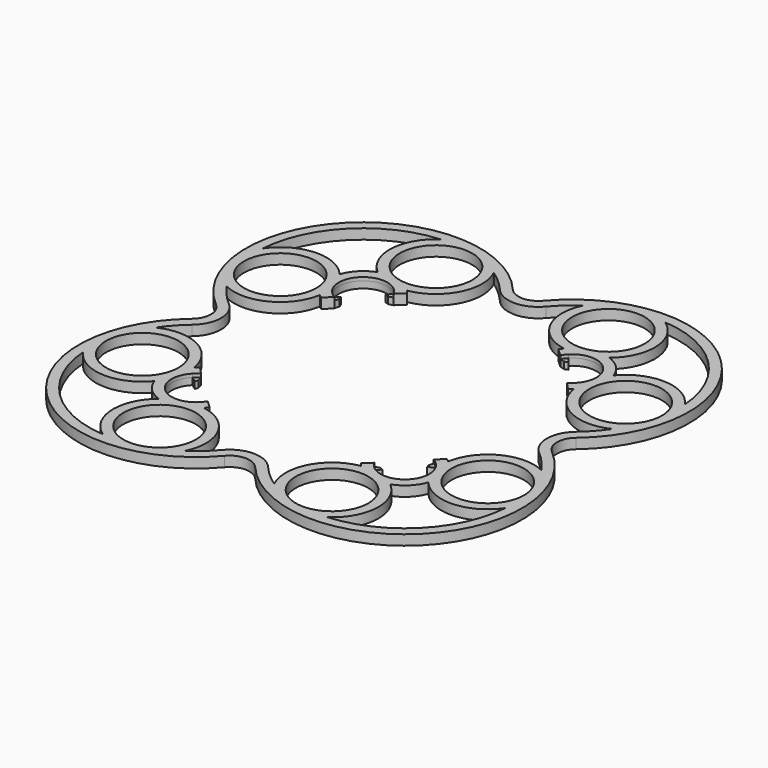
from build123d import *
from build123d import SkipClean  # not in build123d's __all__

# Parameters (mm, degrees)
F1_R     = 5.375
F2_DEPTH = 1.5
F3_R     = 3.6
F4_DEPTH = 0.5


with BuildPart() as f2:
    # F1 (on face) → F2 (new body)
    with BuildSketch(Plane.XY):
        with BuildLine():
            ThreePointArc((2.2559294574, 26.707903259), (0, 25.6616888853), (-2.2559294574, 26.707903259))
            ThreePointArc((-2.2559294574, 26.707903259), (-27.7683026536, 27.7683026536), (-26.707903259, 2.2559294574))
            ThreePointArc((-26.707903259, 2.2559294574), (-25.6616888853, 0), (-26.707903259, -2.2559294574))
            ThreePointArc((-26.707903259, -2.2559294574), (-27.7683026536, -27.7683026536), (-2.2559294574, -26.707903259))
            ThreePointArc((-2.2559294574, -26.707903259), (0, -25.6616888853), (2.2559294574, -26.707903259))
            ThreePointArc((2.2559294574, -26.707903259), (27.7683026536, -27.7683026536), (26.707903259, -2.2559294574))
            ThreePointArc((26.707903259, -2.2559294574), (25.6616888853, 0), (26.707903259, 2.2559294574))
            ThreePointArc((26.707903259, 2.2559294574), (27.7683026536, 27.7683026536), (2.2559294574, 26.707903259))
        make_face()
        with BuildLine():
            ThreePointArc((-20.3191250437, -17.1691416396), (-19.1062445841, -19.1062445841), (-17.1691416396, -20.3191250437))
            ThreePointArc((-17.1691416396, -20.3191250437), (-19.6561239457, -25.9443476809), (-16.6470208781, -31.3084421467))
            ThreePointArc((-16.6470208781, -31.3084421467), (-26.7076424818, -26.7076424818), (-31.3084421467, -16.6470208781))
            ThreePointArc((-31.3084421467, -16.6470208781), (-25.9443476809, -19.6561239457), (-20.3191250437, -17.1691416396))
        make_face(mode=Mode.SUBTRACT)
        with Locations((-12.7888705026, -25.6180730304)):
            Circle(F1_R, mode=Mode.SUBTRACT)
        with Locations((-25.6180730304, -12.7888705026)):
            Circle(F1_R, mode=Mode.SUBTRACT)
        with Locations((12.7888705026, -25.6180730304)):
            Circle(F1_R, mode=Mode.SUBTRACT)
        with BuildLine():
            ThreePointArc((17.1691416396, -20.3191250437), (19.1062445841, -19.1062445841), (20.3191250437, -17.1691416396))
            ThreePointArc((20.3191250437, -17.1691416396), (25.9443476809, -19.6561239457), (31.3084421467, -16.6470208781))
            ThreePointArc((31.3084421467, -16.6470208781), (26.7076424818, -26.7076424818), (16.6470208781, -31.3084421467))
            ThreePointArc((16.6470208781, -31.3084421467), (19.6561239457, -25.9443476809), (17.1691416396, -20.3191250437))
        make_face(mode=Mode.SUBTRACT)
        with Locations((25.6180730304, -12.7888705026)):
            Circle(F1_R, mode=Mode.SUBTRACT)
        with Locations((-25.6180730304, 12.7888705026)):
            Circle(F1_R, mode=Mode.SUBTRACT)
        with BuildLine():
            ThreePointArc((-17.1691416396, 20.3191250437), (-19.1062445841, 19.1062445841), (-20.3191250437, 17.1691416396))
            ThreePointArc((-20.3191250437, 17.1691416396), (-25.9443476809, 19.6561239457), (-31.3084421467, 16.6470208781))
            ThreePointArc((-31.3084421467, 16.6470208781), (-26.7076424818, 26.7076424818), (-16.6470208781, 31.3084421467))
            ThreePointArc((-16.6470208781, 31.3084421467), (-19.6561239457, 25.9443476809), (-17.1691416396, 20.3191250437))
        make_face(mode=Mode.SUBTRACT)
        with Locations((-12.7888705026, 25.6180730304)):
            Circle(F1_R, mode=Mode.SUBTRACT)
        with BuildLine():
            Line((-17.2474476501, 12.3525523499), (-17.0531188132, 13.0769391962))
            Line((-17.0531188132, 13.0769391962), (-17.2364935, 13.5420990873))
            Line((-17.2364935, 13.5420990873), (-18.0455844123, 12.9544155877))
            ThreePointArc((-18.0455844123, 12.9544155877), (-18.0455844123, 18.0455844123), (-12.9544155877, 18.0455844123))
            Line((-12.9544155877, 18.0455844123), (-13.5420990873, 17.2364935))
            Line((-13.5420990873, 17.2364935), (-13.0769391962, 17.0531188132))
            Line((-13.0769391962, 17.0531188132), (-12.3525523499, 17.2474476501))
            Line((-12.3525523499, 17.2474476501), (-11.2336242687, 18.2942866924))
            ThreePointArc((-11.2336242687, 18.2942866924), (-11.4301508715, 18.5734879325), (-11.6449184157, 18.838913892))
            ThreePointArc((-11.6449184157, 18.838913892), (-6.6785172413, 22.4670084448), (-6.6024297076, 28.6170020543))
            ThreePointArc((-6.6024297076, 28.6170020543), (-4.9035215764, 27.2871601762), (-3.4009499654, 25.7389202683))
            ThreePointArc((-3.4009499654, 25.7389202683), (0, 24.1616888853), (3.4009499654, 25.7389202683))
            ThreePointArc((3.4009499654, 25.7389202683), (4.9035215764, 27.2871601762), (6.6024297076, 28.6170020543))
            ThreePointArc((6.6024297076, 28.6170020543), (6.6785172413, 22.4670084448), (11.6449184157, 18.838913892))
            ThreePointArc((11.6449184157, 18.838913892), (11.4301869928, 18.573535763), (11.2336899494, 18.2943869725))
            Line((11.2336899494, 18.2943869725), (12.3525523499, 17.2474476501))
            Line((12.3525523499, 17.2474476501), (13.0769391962, 17.0531188132))
            Line((13.0769391962, 17.0531188132), (13.5420990873, 17.2364935))
            Line((13.5420990873, 17.2364935), (12.9544155877, 18.0455844123))
            ThreePointArc((12.9544155877, 18.0455844123), (18.0455844123, 18.0455844123), (18.0455844123, 12.9544155877))
            Line((18.0455844123, 12.9544155877), (17.2364935, 13.5420990873))
            Line((17.2364935, 13.5420990873), (17.0531188132, 13.0769391962))
            Line((17.0531188132, 13.0769391962), (17.2474476501, 12.3525523499))
            Line((17.2474476501, 12.3525523499), (18.2942866924, 11.2336242687))
            ThreePointArc((18.2942866924, 11.2336242687), (18.5734879325, 11.4301508715), (18.838913892, 11.6449184157))
            ThreePointArc((18.838913892, 11.6449184157), (22.4670084448, 6.6785172413), (28.6170020543, 6.6024297076))
            ThreePointArc((28.6170020543, 6.6024297076), (27.2871601762, 4.9035215764), (25.7389202683, 3.4009499654))
            ThreePointArc((25.7389202683, 3.4009499654), (24.1616888853, 0), (25.7389202683, -3.4009499654))
            ThreePointArc((25.7389202683, -3.4009499654), (27.2871601762, -4.9035215764), (28.6170020543, -6.6024297076))
            ThreePointArc((28.6170020543, -6.6024297076), (22.4670084448, -6.6785172413), (18.838913892, -11.6449184157))
            ThreePointArc((18.838913892, -11.6449184157), (18.573535763, -11.4301869928), (18.2943869725, -11.2336899494))
            Line((18.2943869725, -11.2336899494), (17.2474476501, -12.3525523499))
            Line((17.2474476501, -12.3525523499), (17.0531188132, -13.0769391962))
            Line((17.0531188132, -13.0769391962), (17.2364935, -13.5420990873))
            Line((17.2364935, -13.5420990873), (18.0455844123, -12.9544155877))
            ThreePointArc((18.0455844123, -12.9544155877), (18.0455844123, -18.0455844123), (12.9544155877, -18.0455844123))
            Line((12.9544155877, -18.0455844123), (13.5420990873, -17.2364935))
            Line((13.5420990873, -17.2364935), (13.0769391962, -17.0531188132))
            Line((13.0769391962, -17.0531188132), (12.3525523499, -17.2474476501))
            Line((12.3525523499, -17.2474476501), (11.2336242687, -18.2942866924))
            ThreePointArc((11.2336242687, -18.2942866924), (11.4301508715, -18.5734879325), (11.6449184157, -18.838913892))
            ThreePointArc((11.6449184157, -18.838913892), (6.6785172413, -22.4670084448), (6.6024297076, -28.6170020543))
            ThreePointArc((6.6024297076, -28.6170020543), (4.9035215764, -27.2871601762), (3.4009499654, -25.7389202683))
            ThreePointArc((3.4009499654, -25.7389202683), (0, -24.1616888853), (-3.4009499654, -25.7389202683))
            ThreePointArc((-3.4009499654, -25.7389202683), (-4.9035215764, -27.2871601762), (-6.6024297076, -28.6170020543))
            ThreePointArc((-6.6024297076, -28.6170020543), (-6.6785172413, -22.4670084448), (-11.6449184157, -18.838913892))
            ThreePointArc((-11.6449184157, -18.838913892), (-11.4301869928, -18.573535763), (-11.2336899494, -18.2943869725))
            Line((-11.2336899494, -18.2943869725), (-12.3525523499, -17.2474476501))
            Line((-12.3525523499, -17.2474476501), (-13.0769391962, -17.0531188132))
            Line((-13.0769391962, -17.0531188132), (-13.5420990873, -17.2364935))
            Line((-13.5420990873, -17.2364935), (-12.9544155877, -18.0455844123))
            ThreePointArc((-12.9544155877, -18.0455844123), (-18.0455844123, -18.0455844123), (-18.0455844123, -12.9544155877))
            Line((-18.0455844123, -12.9544155877), (-17.2364935, -13.5420990873))
            Line((-17.2364935, -13.5420990873), (-17.0531188132, -13.0769391962))
            Line((-17.0531188132, -13.0769391962), (-17.2474476501, -12.3525523499))
            Line((-17.2474476501, -12.3525523499), (-18.2942866924, -11.2336242687))
            ThreePointArc((-18.2942866924, -11.2336242687), (-18.5734879325, -11.4301508715), (-18.838913892, -11.6449184157))
            ThreePointArc((-18.838913892, -11.6449184157), (-22.4670084448, -6.6785172413), (-28.6170020543, -6.6024297076))
            ThreePointArc((-28.6170020543, -6.6024297076), (-27.2871601762, -4.9035215764), (-25.7389202683, -3.4009499654))
            ThreePointArc((-25.7389202683, -3.4009499654), (-24.1616888853, 0), (-25.7389202683, 3.4009499654))
            ThreePointArc((-25.7389202683, 3.4009499654), (-27.2871601762, 4.9035215764), (-28.6170020543, 6.6024297076))
            ThreePointArc((-28.6170020543, 6.6024297076), (-22.4670084448, 6.6785172413), (-18.838913892, 11.6449184157))
            ThreePointArc((-18.838913892, 11.6449184157), (-18.573535763, 11.4301869928), (-18.2943869725, 11.2336899494))
            Line((-18.2943869725, 11.2336899494), (-17.2474476501, 12.3525523499))
        make_face(mode=Mode.SUBTRACT)
        with Locations((25.6180730304, 12.7888705026)):
            Circle(F1_R, mode=Mode.SUBTRACT)
        with Locations((12.7888705026, 25.6180730304)):
            Circle(F1_R, mode=Mode.SUBTRACT)
        with BuildLine():
            ThreePointArc((20.3191250437, 17.1691416396), (19.1062445841, 19.1062445841), (17.1691416396, 20.3191250437))
            ThreePointArc((17.1691416396, 20.3191250437), (19.6561239457, 25.9443476809), (16.6470208781, 31.3084421467))
            ThreePointArc((16.6470208781, 31.3084421467), (26.7076424818, 26.7076424818), (31.3084421467, 16.6470208781))
            ThreePointArc((31.3084421467, 16.6470208781), (25.9443476809, 19.6561239457), (20.3191250437, 17.1691416396))
        make_face(mode=Mode.SUBTRACT)
    extrude(amount=F2_DEPTH)

    # F3 (on face) → F4 (cut)
    with BuildSketch(Plane.XY.offset(1.5)):
        with Locations((-15.5, 15.5)):
            Circle(F3_R)
        with Locations((-15.5, -15.5)):
            Circle(F3_R)
        with Locations((15.5, -15.5)):
            Circle(F3_R)
        with Locations((15.5, 15.5)):
            Circle(F3_R)
    with SkipClean():  # cleaning this boolean's faces spoils the solid; the shape is the same uncleaned
        extrude(amount=-F4_DEPTH, mode=Mode.SUBTRACT)


solid = f2.part
